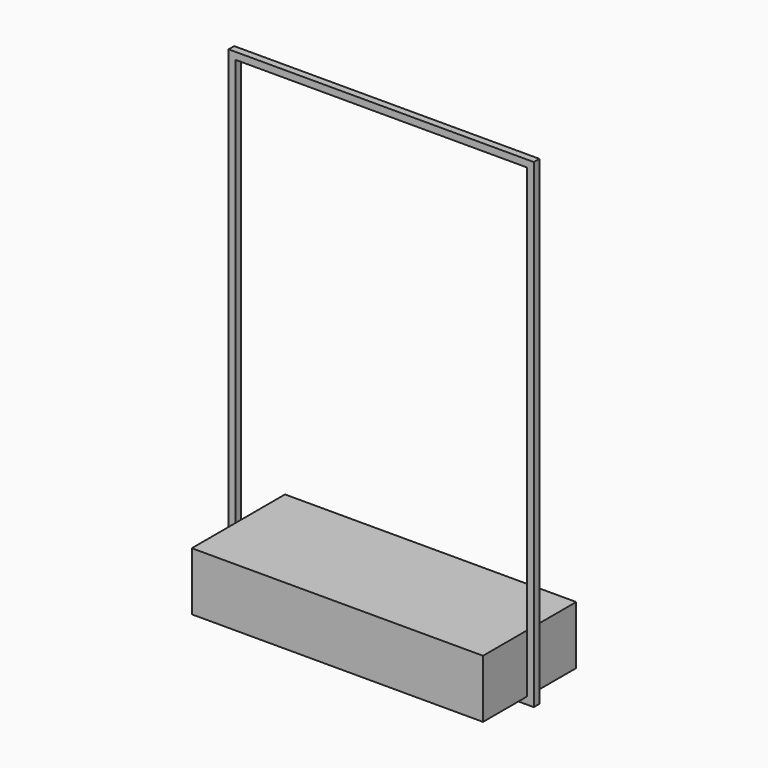
from build123d import *

# Parameters (mm, degrees)
F0_W     = 1250
F0_H     = 500
F1_DEPTH = 250
F2_W     = 1310
F2_H     = 2060
F2_W_2   = 1250
F2_H_2   = 2000
F3_DEPTH = 15
F4_W     = 1050
F4_H     = 300
F4_W_2   = 990
F4_H_2   = 240
F5_DEPTH = 30


with BuildPart() as f1:
    # F0 (on Top) → F1 (new body)
    with BuildSketch(Plane.XY):
        Rectangle(F0_W, F0_H)
    extrude(amount=F1_DEPTH)


with BuildPart() as f3:
    # F2 (on Front) → F3 (new body, symmetric)
    with BuildSketch(Plane.XZ):
        with Locations((0, 1000)):
            Rectangle(F2_W, F2_H)
        with Locations((0, 1000)):
            Rectangle(F2_W_2, F2_H_2, mode=Mode.SUBTRACT)
    extrude(amount=F3_DEPTH, both=True)

    # F4 (on face) → F5 (join)
    with BuildSketch(Plane(origin=(0, 0, 0), x_dir=(1, 0, 0), z_dir=(0, 0, -1))):
        Rectangle(F4_W, F4_H)
        Rectangle(F4_W_2, F4_H_2, mode=Mode.SUBTRACT)
    extrude(amount=F5_DEPTH)


solid = Compound([f1.part, f3.part])
